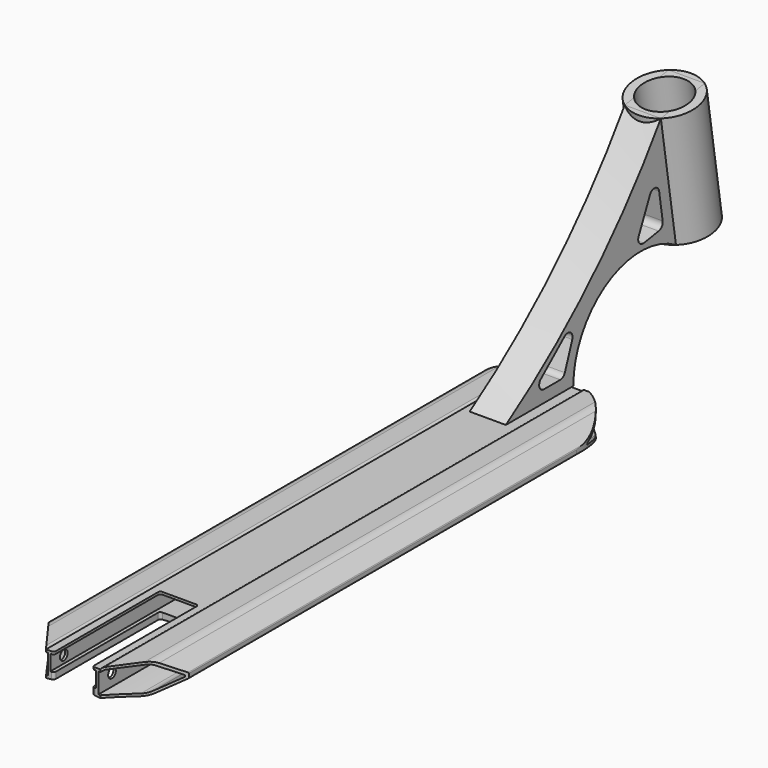
from build123d import *

# Parameters (mm, degrees)
F1_DEPTH    = 250
F2_W        = 38
F2_H        = 13
F3_DEPTH    = 500.001
F4_T1_DEPTH = 509.3674969976
F5_R        = 9
F6_R        = 1
F8_DEPTH    = 500.001
F9_DEPTH    = 500.0010001
F11_DEPTH   = 50
F13_DEPTH   = 24.8040289874
F14_R       = 2
F16_DEPTH   = 15
F17_R       = 27.459
F18_DEPTH   = 100
F20_D       = 40
F22_D       = 8
F24_DEPTH   = 115.0010001
F25_R       = 5


# Not quite as in the source:
# - a fillet or chamfer that OpenCascade refuses, or shapes differently, is made with other operations: its cross-section is extruded or revolved along the edge and cut away or added
# - ends of sketch curves that miss each other by under 0.0002 mm in the source are joined


with BuildPart() as f1:
    # F0 (on Front) → F1 (new body, symmetric)
    with BuildSketch(Plane.XZ):
        with BuildLine():
            Line((22.5, 10.6806829985), (0, 10.6806829985))
            Line((0, 10.6806829985), (-22.5, 10.6806829985))
            Line((-22.5, 10.6806829985), (-22.5, 11.9806829985))
            Line((-22.5, 11.9806829985), (-43.2219779947, 11.9806829985))
            Line((-43.2219779947, 11.9806829985), (-57.5, 0))
            Line((-57.5, 0), (-57.5, -4))
            Line((-57.5, -4), (-41.3584694616, -13.3193170015))
            ThreePointArc((-41.3584694616, -13.3193170015), (0, -8.9962880629), (41.3584694616, -13.3193170015))
            Line((41.3584694616, -13.3193170015), (57.5, -4))
            Line((57.5, -4), (57.5, 0))
            Line((57.5, 0), (43.2219779947, 11.9806829985))
            Line((43.2219779947, 11.9806829985), (22.5, 11.9806829985))
            Line((22.5, 11.9806829985), (22.5, 10.6806829985))
        make_face()
    extrude(amount=F1_DEPTH, both=True)

    # F2 (on face) → F3 (cut, through all)
    with BuildSketch(Plane.XZ.offset(250)):
        with Locations((0, 2.1806829985)):
            Rectangle(F2_W, F2_H)
    extrude(amount=-F3_DEPTH, mode=Mode.SUBTRACT)

    # F4: fillet of radius 2 on 2 edges, made by hand

    # F4_s2 → F4_t1 (cut)
    with BuildSketch(Plane.XZ.offset(-254.6837484988)):
        with BuildLine():
            ThreePointArc((-24.3734993995, 11.9806829985), (-23.2333239744, 11.6238506711), (-22.5, 10.6806829985))
            Line((-22.5, 10.6806829985), (-22.5, 11.9806829985))
            Line((-22.5, 11.9806829985), (-24.3734993995, 11.9806829985))
        make_face()
        with BuildLine():
            ThreePointArc((24.3734993995, 11.9806829985), (23.2333239744, 11.6238506711), (22.5, 10.6806829985))
            Line((22.5, 10.6806829985), (22.5, 11.9806829985))
            Line((22.5, 11.9806829985), (24.3734993995, 11.9806829985))
        make_face()
    extrude(amount=F4_T1_DEPTH, mode=Mode.SUBTRACT)

    # F5
    f5_edges = [f1.edges().sort_by_distance(p)[0] for p in [
        (-41.358469, 0, -13.319317),
        (41.358469, 0, -13.319317),
        (-43.221978, 0, 11.980683),
        (43.221978, 0, 11.980683),
    ]]
    fillet(f5_edges, radius=F5_R)

    # F6
    f6_edges = [f1.edges().sort_by_distance(p)[0] for p in [
        (57.5, 0, 0),
        (57.5, 0, -4),
        (-57.5, 0, 0),
        (-57.5, 0, -4),
    ]]
    fillet(f6_edges, radius=F6_R)

    # F7 (on face) → F8 (cut, through all)
    with BuildSketch(Plane.XZ.offset(250)):
        with BuildLine():
            Line((-21, -8.0908375728), (-21, 8.6806826293))
            Line((-21, 8.6806826293), (-22.5, 8.6806826293))
            add(Edge.make_bspline(
                [(-23.1244997998, 9.1140161579), (-22.9163331999, 8.9695716484), (-22.7081665999, 8.8251271389), (-22.5, 8.6806826293)],
                knots=[1.5202341227, 1.5202341227, 1.5202341227, 1.5202341227, 2.2803511841, 2.2803511841, 2.2803511841, 2.2803511841], degree=3))
            add(Edge.make_bspline(
                [(-23.1244997998, 9.1140161579), (-23.2417391466, 9.1953672485), (-23.3589784934, 9.2767183392), (-23.4762178402, 9.3580694298)],
                knots=[0, 0, 0, 0, 0.4280976284, 0.4280976284, 0.4280976284, 0.4280976284], degree=3))
            add(Edge.make_bspline(
                [(-24.3734993995, 9.980683215), (-24.0744055464, 9.7731452866), (-23.7753116933, 9.5656073582), (-23.4762178402, 9.3580694298)],
                knots=[0, 0, 0, 0, 1.0921364943, 1.0921364943, 1.0921364943, 1.0921364943], degree=3))
            Line((-24.3734993995, 9.980683215), (-39.9462458864, 9.980683215))
            ThreePointArc((-39.9462458864, 9.980683215), (-42.340386903, 9.5585313809), (-44.4457591794, 8.3429941304))
            Line((-44.4457591794, 8.3429941304), (-55.8571735331, -1.232319445))
            Line((-55.8571735331, -1.232319445), (-55.9999666626, -2.5566434697))
            Line((-55.9999666626, -2.5566434697), (-43.3077059014, -9.8845236368))
            ThreePointArc((-43.3077059014, -9.8845236368), (-40.9642400468, -10.7261439454), (-38.474433516, -10.6942003224))
            ThreePointArc((-38.474433516, -10.6942003224), (-29.7656922465, -9.2013842197), (-21, -8.0908375728))
        make_face()
        with BuildLine():
            Line((22.5, 8.6806826293), (21, 8.6806826293))
            Line((21, 8.6806826293), (21, -8.0908375728))
            ThreePointArc((21, -8.0908375728), (29.7656922465, -9.2013842197), (38.474433516, -10.6942003224))
            ThreePointArc((38.474433516, -10.6942003224), (40.9642400468, -10.7261439454), (43.3077059014, -9.8845236368))
            Line((43.3077059014, -9.8845236368), (55.9999666626, -2.5566434697))
            Line((55.9999666626, -2.5566434697), (55.8571735331, -1.232319445))
            Line((55.8571735331, -1.232319445), (44.4457591794, 8.3429941304))
            ThreePointArc((44.4457591794, 8.3429941304), (42.340386903, 9.5585313809), (39.9462458864, 9.9806830378))
            Line((39.9462458864, 9.9806830378), (24.3734993995, 9.980683215))
            Line((24.3734993995, 9.980683215), (22.5, 8.6806826293))
        make_face()
    extrude(amount=-F8_DEPTH, mode=Mode.SUBTRACT)

    # F7 (on face) → F9 (cut, through all)
    with BuildSketch(Plane.XZ.offset(250)):
        with BuildLine():
            Line((-21, -8.0908375728), (-21, 8.6806826293))
            Line((-21, 8.6806826293), (-22.5, 8.6806826293))
            add(Edge.make_bspline(
                [(-23.1244997998, 9.1140161579), (-22.9163331999, 8.9695716484), (-22.7081665999, 8.8251271389), (-22.5, 8.6806826293)],
                knots=[1.5202341227, 1.5202341227, 1.5202341227, 1.5202341227, 2.2803511841, 2.2803511841, 2.2803511841, 2.2803511841], degree=3))
            add(Edge.make_bspline(
                [(-23.1244997998, 9.1140161579), (-23.2417391466, 9.1953672485), (-23.3589784934, 9.2767183392), (-23.4762178402, 9.3580694298)],
                knots=[0, 0, 0, 0, 0.4280976284, 0.4280976284, 0.4280976284, 0.4280976284], degree=3))
            add(Edge.make_bspline(
                [(-24.3734993995, 9.980683215), (-24.0744055464, 9.7731452866), (-23.7753116933, 9.5656073582), (-23.4762178402, 9.3580694298)],
                knots=[0, 0, 0, 0, 1.0921364943, 1.0921364943, 1.0921364943, 1.0921364943], degree=3))
            Line((-24.3734993995, 9.980683215), (-39.9462458864, 9.980683215))
            ThreePointArc((-39.9462458864, 9.980683215), (-42.340386903, 9.5585313809), (-44.4457591794, 8.3429941304))
            Line((-44.4457591794, 8.3429941304), (-55.8571735331, -1.232319445))
            Line((-55.8571735331, -1.232319445), (-55.9999666626, -2.5566434697))
            Line((-55.9999666626, -2.5566434697), (-43.3077059014, -9.8845236368))
            ThreePointArc((-43.3077059014, -9.8845236368), (-40.9642400468, -10.7261439454), (-38.474433516, -10.6942003224))
            ThreePointArc((-38.474433516, -10.6942003224), (-29.7656922465, -9.2013842197), (-21, -8.0908375728))
        make_face()
        with BuildLine():
            Line((22.5, 8.6806826293), (21, 8.6806826293))
            Line((21, 8.6806826293), (21, -8.0908375728))
            ThreePointArc((21, -8.0908375728), (29.7656922465, -9.2013842197), (38.474433516, -10.6942003224))
            ThreePointArc((38.474433516, -10.6942003224), (40.9642400468, -10.7261439454), (43.3077059014, -9.8845236368))
            Line((43.3077059014, -9.8845236368), (55.9999666626, -2.5566434697))
            Line((55.9999666626, -2.5566434697), (55.8571735331, -1.232319445))
            Line((55.8571735331, -1.232319445), (44.4457591794, 8.3429941304))
            ThreePointArc((44.4457591794, 8.3429941304), (42.340386903, 9.5585313809), (39.9462458864, 9.9806830378))
            Line((39.9462458864, 9.9806830378), (24.3734993995, 9.980683215))
            Line((24.3734993995, 9.980683215), (22.5, 8.6806826293))
        make_face()
    extrude(amount=-F9_DEPTH, mode=Mode.SUBTRACT)

    # F10 (on face) → F11 (cut, symmetric)
    with BuildSketch(Plane.XY.offset(10.6806829985)):
        with BuildLine():
            ThreePointArc((-57.5, 200), (0, 257.5), (57.5, 200))
            Line((57.5, 200), (57.5, 280))
            Line((57.5, 280), (-57.5, 280))
            Line((-57.5, 280), (-57.5, 200))
        make_face()
    extrude(amount=F11_DEPTH, both=True, mode=Mode.SUBTRACT)

    # F12 (on face) → F13 (cut, through all)
    with BuildSketch(Plane.XY.offset(11.9806829985)):
        Polygon((-22.5, -250), (-68, -187.3746226186), (-68, -287.3746226186), (68, -287.3746226186), (68, -187.3746226186), (22.5, -250), (16, -250), (16, -140), (-16, -140), (-16, -250), align=None)
    extrude(amount=-F13_DEPTH, mode=Mode.SUBTRACT)

    # F14
    f14_edges = [f1.edges().sort_by_distance(p)[0] for p in [
        (-16, -250, 9.680683),
        (-16, -250, -6.978316),
        (-16, -140, -6.978316),
        (-16, -140, 9.680683),
        (16, -250, -6.978316),
        (16, -250, 9.680683),
        (16, -140, -6.978316),
        (16, -140, 9.680683),
    ]]
    fillet(f14_edges, radius=F14_R)

    # F22 (through all)
    with Locations(Plane.YZ.offset(21)):
        with Locations((-236, 1.9091624272)):
            Hole(F22_D / 2)


with BuildPart() as f16:
    # F15 (on Right) → F16 (new body, symmetric)
    with BuildSketch(Plane.YZ):
        with BuildLine():
            ThreePointArc((340.7970211938, 170.5165005353), (268.6221397132, 82.9076686503), (180, 11.9806829985))
            Line((180, 11.9806829985), (250, 11.9806829985))
            ThreePointArc((250, 11.9806829985), (285.7278009084, 73.0168720131), (356.4404676978, 71.7476664758))
            Line((356.4404676978, 71.7476664758), (401.8741313652, 78.9436518676))
            Line((401.8741313652, 78.9436518676), (386.2306848612, 177.7124859271))
            Line((386.2306848612, 177.7124859271), (340.7970211938, 170.5165005353))
        make_face()
    extrude(amount=F16_DEPTH, both=True)

    # F17 (on face) → F18 (join, through all)
    with BuildSketch(Plane(origin=(0, -18.0063515166, 113.687629162), x_dir=(1, 0, 0), z_dir=(0, -0.156434465, 0.9876883406))):
        with Locations((0, 386.2759018844)):
            Circle(F17_R)
    extrude(amount=-F18_DEPTH)

    # F20 (through all)
    with Locations(Plane(origin=(0, -18.0063515166, 113.687629162), x_dir=(1, 0, 0), z_dir=(0, -0.156434465, 0.9876883406))):
        with Locations((0, 386.2759018844)):
            Hole(F20_D / 2)

    # F23 (on face) → F24 (cut, through all)
    with BuildSketch(Plane.YZ.offset(57.5)):
        Polygon((255.3909064497, 64.2668509339), (206, 21.9806829985), (240, 21.9806829985), align=None)
        Polygon((343.434966255, 89.9370999244), (336.3954153282, 134.3830752512), (313.8043160372, 85.2440659732), align=None)
    extrude(amount=-F24_DEPTH, mode=Mode.SUBTRACT)

    # F25
    f25_edges = [f16.edges().sort_by_distance(p)[0] for p in [
        (0, 343.434966, 89.9371),
        (0, 240, 21.980683),
        (0, 255.390906, 64.266851),
        (0, 336.395415, 134.383075),
        (0, 313.804316, 85.244066),
        (0, 206, 21.980683),
    ]]
    fillet(f25_edges, radius=F25_R)


solid = Compound([f1.part, f16.part])
